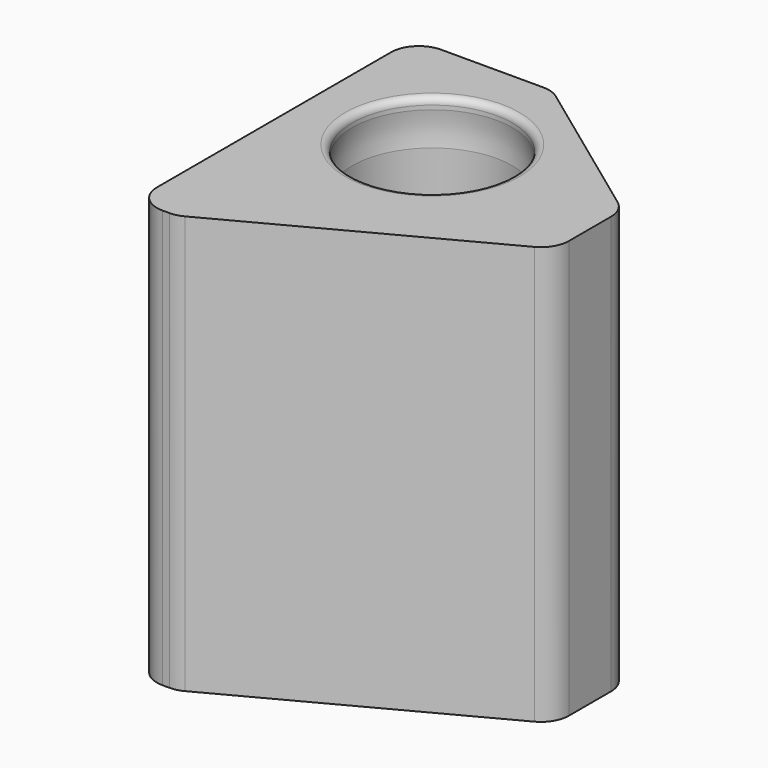
from build123d import *

# Parameters (mm, degrees)
F0_R     = 5.75
F1_DEPTH = 30
F2_R     = 2
F5_R     = 0.5


with BuildPart() as f1:
    # F0 (on Top) → F1 (new body)
    with BuildSketch(Plane.XY):
        Polygon((-8.8044720603, 9.3002779725), (-8.8044720603, -15.6997220275), (-5.8044720603, -15.6997220275), (13.2937646807, -5.5672283149), (13.2937646807, 0.4327716851), (1.1955279397, 9.3002779725), align=None)
        Circle(F0_R, mode=Mode.SUBTRACT)
    extrude(amount=-F1_DEPTH)

    # F2
    f2_edges = [f1.edges().sort_by_distance(p)[0] for p in [
        (-8.804472, 9.300278, -15),
        (1.195528, 9.300278, -15),
        (-8.804472, -15.699722, -15),
        (13.293765, -5.567228, -15),
        (-5.804472, -15.699722, -15),
        (13.293765, 0.432772, -15),
    ]]
    fillet(f2_edges, radius=F2_R)

    # F3 (on Right) → F4 (revolve, cut)
    with BuildSketch(Plane.YZ):
        with BuildLine():
            Line((0, 0), (-5.5240949485, 0))
            ThreePointArc((-5.5240949485, 0), (-4.8096582519, -5.3738423941), (0, -7.875))
            Line((0, -7.875), (0, 0))
        make_face()
    revolve(axis=Axis((0, 0, -1), (0, 0, -1)), mode=Mode.SUBTRACT)

    # F5
    f5_edges = [f1.edges().sort_by_distance(p)[0] for p in [
        (-5.75, 0, 0),
    ]]
    fillet(f5_edges, radius=F5_R)


solid = f1.part
